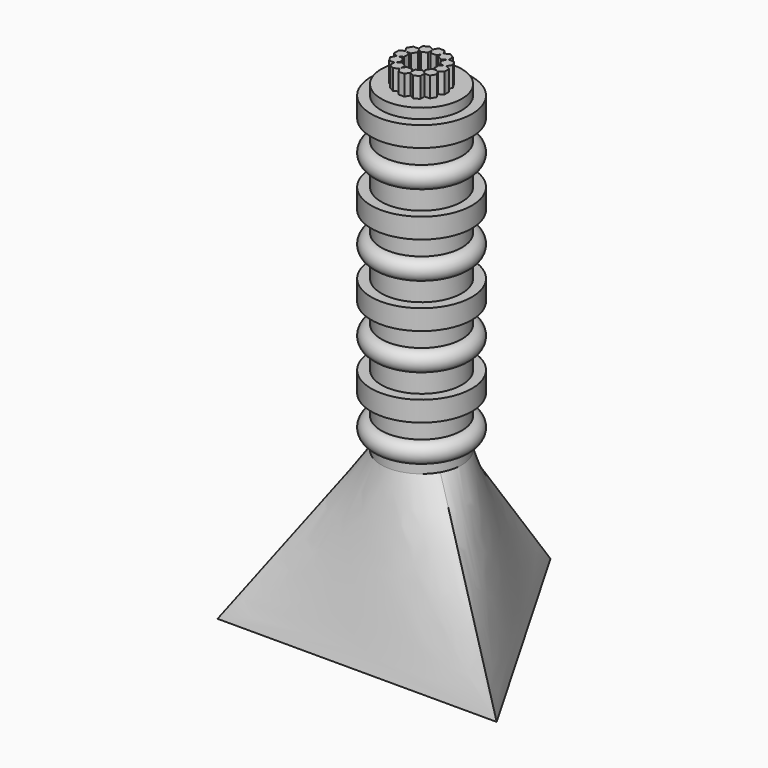
from build123d import *

# Parameters (mm, degrees)
F7_DEPTH = 6.35
F8_COUNT = 12


# Not quite as in the source:
# - the arcs of a loft's sections are written as splines that run evenly, so that the points pair up as in the source's solid


with BuildPart() as f5:
    # F0 (on Front) → F5 (revolve)
    with BuildSketch(Plane.XZ):
        with BuildLine():
            Line((12.7, 47.625), (12.7, 50.8))
            Line((12.7, 50.8), (0, 50.8))
            Line((0, 50.8), (0, -50.8))
            Line((0, -50.8), (12.7, -50.8))
            Line((12.7, -50.8), (12.7, -47.625))
            ThreePointArc((12.7, -47.625), (15.875, -44.45), (12.7, -41.275))
            Line((12.7, -41.275), (12.7, -34.925))
            Line((12.7, -34.925), (15.875, -34.925))
            Line((15.875, -34.925), (15.875, -28.575))
            Line((15.875, -28.575), (12.7, -28.575))
            Line((12.7, -28.575), (12.7, -25.4))
            Line((12.7, -25.4), (12.7, -22.225))
            ThreePointArc((12.7, -22.225), (15.875, -19.05), (12.7, -15.875))
            Line((12.7, -15.875), (12.7, -9.525))
            Line((12.7, -9.525), (15.875, -9.525))
            Line((15.875, -9.525), (15.875, -3.175))
            Line((15.875, -3.175), (12.7, -3.175))
            Line((12.7, -3.175), (12.7, 0))
            Line((12.7, 0), (12.7, 3.175))
            ThreePointArc((12.7, 3.175), (15.875, 6.35), (12.7, 9.525))
            Line((12.7, 9.525), (12.7, 15.875))
            Line((12.7, 15.875), (15.875, 15.875))
            Line((15.875, 15.875), (15.875, 22.225))
            Line((15.875, 22.225), (12.7, 22.225))
            Line((12.7, 22.225), (12.7, 25.4))
            Line((12.7, 25.4), (12.7, 28.575))
            ThreePointArc((12.7, 28.575), (15.875, 31.75), (12.7, 34.925))
            Line((12.7, 34.925), (12.7, 41.275))
            Line((12.7, 41.275), (15.875, 41.275))
            Line((15.875, 41.275), (15.875, 47.625))
            Line((15.875, 47.625), (12.7, 47.625))
        make_face()
    revolve(axis=Axis((0, 0, 0), (0, 0, -1)))

    # F2 (on offset) → F6 section 0
    with BuildSketch(Plane.XY.offset(-101.6)):
        Polygon((-43.9940905122, -25.4), (43.9940905122, -25.4), (0, 50.8), align=None)
    # F5_face (on face) → F6 section 1
    with BuildSketch(Plane(origin=(0, 0, -50.8), x_dir=(1, 0, 0), z_dir=(0, 0, -1))):
        with BuildLine():
            add(Edge.make_bspline(
                [(-10.9985226281, 6.35), (-11.7373786781, 5.0702637819), (-12.25045645, 3.6605941892), (-12.7636604765, 0.7500695235), (-12.7636604765, -0.7500695235), (-12.25045645, -3.6605941892), (-11.7373786781, -5.0702637819), (-10.2596665781, -7.6297362181), (-9.2953957858, -8.778909399), (-7.0314095003, -10.6786194562), (-5.7322509763, -11.4286889797), (-2.9550606642, -12.4395035882), (-1.4777121, -12.7), (0, -12.7)],
                knots=[0, 0, 0, 0, 0.1666666667, 0.1666666667, 0.3333333333, 0.3333333333, 0.5, 0.5, 0.6666666667, 0.6666666667, 0.8333333333, 0.8333333333, 1, 1, 1, 1], degree=3))
            add(Edge.make_bspline(
                [(0, -12.7), (1.4777121, -12.7), (2.9550606642, -12.4395035882), (5.7322509763, -11.4286889797), (7.0314095003, -10.6786194562), (9.2953957858, -8.778909399), (10.2596665781, -7.6297362181), (11.7373786781, -5.0702637819), (12.25045645, -3.6605941892), (12.7636604765, -0.7500695235), (12.7636604765, 0.7500695235), (12.25045645, 3.6605941892), (11.7373786781, 5.0702637819), (10.9985226281, 6.35)],
                knots=[0, 0, 0, 0, 0.1666666667, 0.1666666667, 0.3333333333, 0.3333333333, 0.5, 0.5, 0.6666666667, 0.6666666667, 0.8333333333, 0.8333333333, 1, 1, 1, 1], degree=3))
            add(Edge.make_bspline(
                [(10.9985226281, 6.35), (10.2596665781, 7.6297362181), (9.2953957858, 8.778909399), (7.0314095003, 10.6786194562), (5.7322509763, 11.4286889797), (2.9550606642, 12.4395035882), (1.4777121, 12.7), (-1.4777121, 12.7), (-2.9550606642, 12.4395035882), (-5.7322509763, 11.4286889797), (-7.0314095003, 10.6786194562), (-9.2953957858, 8.778909399), (-10.2596665781, 7.6297362181), (-10.9985226281, 6.35)],
                knots=[0, 0, 0, 0, 0.1666666667, 0.1666666667, 0.3333333333, 0.3333333333, 0.5, 0.5, 0.6666666667, 0.6666666667, 0.8333333333, 0.8333333333, 1, 1, 1, 1], degree=3))
        make_face()
    loft(ruled=True)



with BuildPart() as f7:
    # F4 (on offset) → F7 (new body)
    with BuildSketch(Plane.XY.offset(50.8)):
        Polygon((-4.7625, -0.9165435523), (-4.7625, 0.9165435523), (-6.35, 1.8330871047), (-7.9375, 0.9165435523), (-7.9375, -0.9165435523), (-6.35, -1.8330871047), align=None)
    extrude(amount=F7_DEPTH)


with BuildPart() as f5_1:
    add(f5.part)

    add(f7.part)  # F8 merges F7
    # F8: F7 ×12 about axis
    f8_axis = Axis((0, 0, 47.625), (0, 0, -1))
    for i in range(1, F8_COUNT):
        add(f7.part.rotate(f8_axis, i * 360 / F8_COUNT))


solid = f5_1.part
